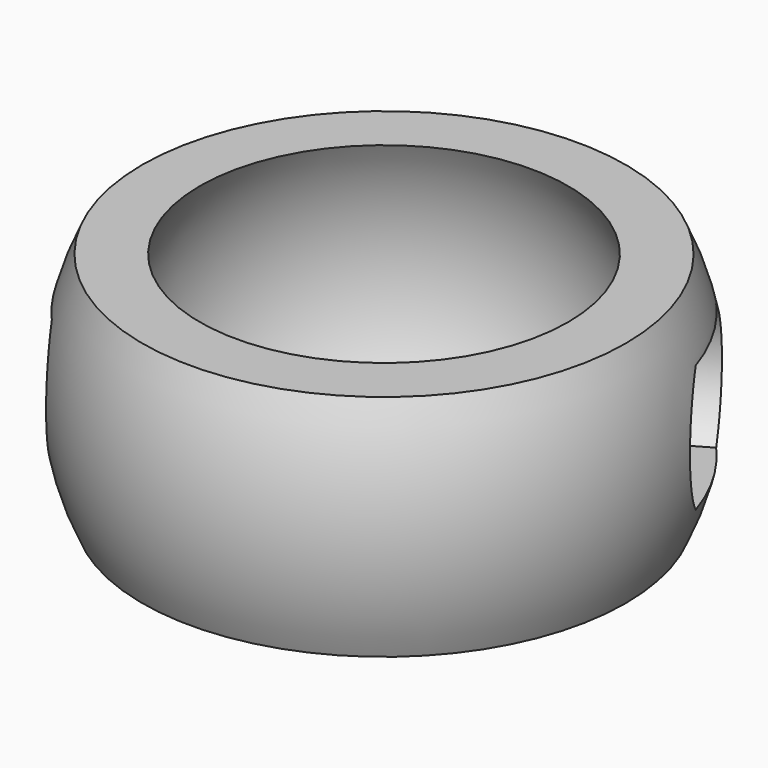
from build123d import *

# Parameters (mm, degrees)
F5_DEPTH = 12.7


# Not quite as in the source:
# - a pattern or mirror of a feature is missing from the dataset's text; its kind, count and spacing are read off the source's solid


with BuildPart() as f1:
    # F0 (on Front) → F1 (revolve)
    with BuildSketch(Plane.XZ):
        with BuildLine():
            ThreePointArc((-23.0108623865, -28.5877), (-27.0923504321, -14.2949750325), (-23.01875, 0))
            Line((-23.01875, 0), (-30.2104195144, 0))
            ThreePointArc((-30.2104195144, 0), (-33.4185884522, -14.2945250314), (-30.20441, -28.5877))
            Line((-30.20441, -28.5877), (-23.0108623865, -28.5877))
        make_face()
    revolve(axis=Axis((0, 0, -13.0283376202), (0, 0, -1)))

    # F4 (on line) → F5 (cut)
    with BuildSketch(Plane(origin=(28.9413471977, 16.7092945953, 0), x_dir=(-0.5, 0.8660254038, 0), z_dir=(0.8660254038, 0.5, 0))):
        with BuildLine():
            Line((-6.6390036837, -22.225), (6.6390036837, -22.225))
            ThreePointArc((6.6390036837, -22.225), (10.34796, -14.2875), (6.6390036837, -6.35))
            Line((6.6390036837, -6.35), (-6.6390036837, -6.35))
            ThreePointArc((-6.6390036837, -6.35), (-10.34796, -14.2875), (-6.6390036837, -22.225))
        make_face()
    f5 = extrude(amount=-F5_DEPTH, mode=Mode.SUBTRACT)

    # F5_copies: F5 across plane
    add(f5.mirror(Plane(origin=(0, 0, 0), x_dir=(0.5, -0.8660254038, 0), z_dir=(-0.8660254038, -0.5, 0))), mode=Mode.SUBTRACT)


solid = f1.part
